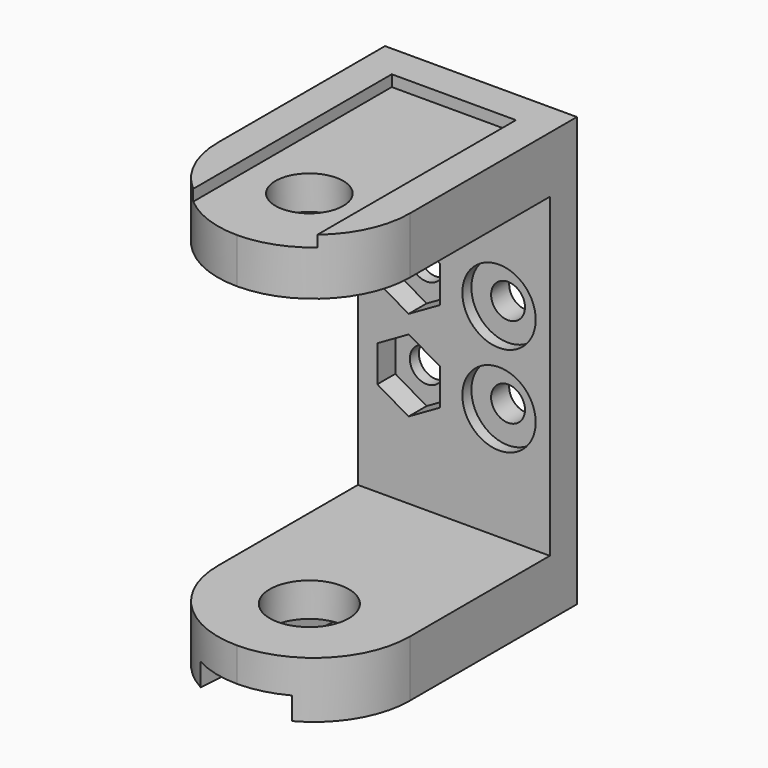
from build123d import *

# Parameters (mm, degrees)
F0_W            = 17
F0_H            = 38
F1_DEPTH        = 3
F2_W            = 17
F2_H            = 5
F3_DEPTH        = 24
F4_R            = 8.49999
F5_R            = 3
F6_DEPTH        = 40
F7_W            = 11
F7_H            = 29.9753743202
F8_DEPTH        = 1
F10_DEPTH       = 2
F11_R           = 5.5
F12_DEPTH       = 1
F14_D           = 1
F14_DEPTH       = 20
F14_TIP         = 0.3004303095
F16_D           = 3
F16_DEPTH       = 20
F16_CBORE_D     = 6.5
F16_CBORE_DEPTH = 1
F16_TIP         = 0.9012909285
F18_R           = 3.5
F19_DEPTH       = 25
F21_DEPTH       = 2
F22_D           = 3


# Not quite as in the source:
# - a fillet or chamfer is up to 0.001 mm smaller than in the source, because OpenCascade refuses the exact size
# - a feature names something its author has since deleted; it is built from what else it names


with BuildPart() as f1:
    # F0 (on Front) → F1 (new body)
    with BuildSketch(Plane.XZ):
        Rectangle(F0_W, F0_H)
    extrude(amount=F1_DEPTH)

    # F2 (on face) → F3 (join)
    with BuildSketch(Plane.XZ.offset(3)):
        with Locations((0, -16.5)):
            Rectangle(F2_W, F2_H)
        with Locations((0, 16.5)):
            Rectangle(F2_W, F2_H)
    extrude(amount=F3_DEPTH)

    # F4 (radius 8.5 in the source; OpenCascade refuses exactly that, so slightly less here)
    f4_edges = [f1.edges().sort_by_distance(p)[0] for p in [
        (8.5, -27, -16.5),
        (-8.5, -27, -16.5),
        (8.5, -27, 16.5),
        (-8.5, -27, 16.5),
    ]]
    fillet(f4_edges, radius=F4_R)

    # F5 (on face) → F6 (cut)
    with BuildSketch(Plane(origin=(0, 0, -19), x_dir=(1, 0, 0), z_dir=(0, 0, -1))):
        with Locations((0, 19)):
            Circle(F5_R)
    extrude(amount=-F6_DEPTH, mode=Mode.SUBTRACT)

    # F7 (on face) → F8 (cut)
    with BuildSketch(Plane.XY.offset(19)):
        with Locations((0, -17.9876871601)):
            Rectangle(F7_W, F7_H)
    extrude(amount=-F8_DEPTH, mode=Mode.SUBTRACT)

    # F9 (on face) → F10 (cut)
    with BuildSketch(Plane(origin=(0, 0, -19), x_dir=(1, 0, 0), z_dir=(0, 0, -1))):
        with BuildLine():
            Line((4.2340652424, 28.3797578726), (-4.2340652424, 28.3797578726))
            Line((-4.2340652424, 28.3797578726), (-3.4896296074, 18.730769238))
            ThreePointArc((-3.4896296074, 18.730769238), (-0.1347152072, 22.4974064409), (3.5, 19))
            ThreePointArc((3.5, 19), (3.4974064409, 18.8652847928), (3.4896296074, 18.730769238))
            Line((3.4896296074, 18.730769238), (4.2340652424, 28.3797578726))
        make_face()
        with BuildLine():
            ThreePointArc((3.4896296074, 18.730769238), (0, 15.5), (-3.4896296074, 18.730769238))
            Line((-3.4896296074, 18.730769238), (-2.4925925763, 5.8076923077))
            ThreePointArc((-2.4925925763, 5.8076923077), (0, 3.5), (2.4925925763, 5.8076923077))
            Line((2.4925925763, 5.8076923077), (3.4896296074, 18.730769238))
        make_face()
        with BuildLine():
            ThreePointArc((3.5, 19), (-0.1347152072, 22.4974064409), (-3.4896296074, 18.730769238))
            ThreePointArc((-3.4896296074, 18.730769238), (0, 15.5), (3.4896296074, 18.730769238))
            ThreePointArc((3.4896296074, 18.730769238), (3.4974064409, 18.8652847928), (3.5, 19))
        make_face()
    extrude(amount=-F10_DEPTH, mode=Mode.SUBTRACT)

    # F11 (on face) → F12 (cut)
    with BuildSketch(Plane(origin=(0, 0, 14), x_dir=(1, 0, 0), z_dir=(0, 0, -1))):
        with Locations((0, 19)):
            Circle(F11_R)
    extrude(amount=-F12_DEPTH, mode=Mode.SUBTRACT)

    # F14
    with Locations(Plane(origin=(0, 0, 0), x_dir=(-1, 0, 0), z_dir=(0, 1, 0))):
        with Locations((-4, 4), (-4, -4)):
            Hole(F14_D / 2, depth=F14_DEPTH)
            with Locations((0, 0, -(F14_DEPTH + F14_TIP / 2))):  # 118° drill point
                Cone(0, F14_D / 2, F14_TIP, mode=Mode.SUBTRACT)

    # F16
    with Locations(Plane.XZ.offset(3)):
        with Locations((4, 4), (4, -4)):
            CounterBoreHole(F16_D / 2, F16_CBORE_D / 2, F16_CBORE_DEPTH, depth=F16_DEPTH)
            with Locations((0, 0, -(F16_DEPTH + F16_TIP / 2))):  # 118° drill point
                Cone(0, F16_D / 2, F16_TIP, mode=Mode.SUBTRACT)

    # F18 (on face) → F19 (cut)
    with BuildSketch(Plane(origin=(0, 0, -17), x_dir=(1, 0, 0), z_dir=(0, 0, -1))):
        with Locations((0, 19)):
            Circle(F18_R)
    extrude(amount=-F19_DEPTH, mode=Mode.SUBTRACT)

    # F20 (on face) → F21 (cut)
    with BuildSketch(Plane.XZ.offset(3)):
        Polygon((-1.2190877389, 5.5914901538), (-3.9878147725, 7.2040857407), (-6.7687270336, 5.6125955869), (-6.7809122611, 2.4085098462), (-4.0121852275, 0.7959142593), (-1.2312729664, 2.3874044131), align=None)
        Polygon((-1.2179301405, -2.4078473634), (-3.9878097002, -0.7945805083), (-6.7698795597, -2.3867331448), (-6.7820698595, -5.5921526366), (-4.0121902998, -7.2054194917), (-1.2301204403, -5.6132668552), align=None)
    extrude(amount=-F21_DEPTH, mode=Mode.SUBTRACT)

    # F22 (through all)
    with Locations(Plane.XZ.offset(3)):
        with Locations((-4, 4), (-4, -4)):
            Hole(F22_D / 2)


solid = f1.part
